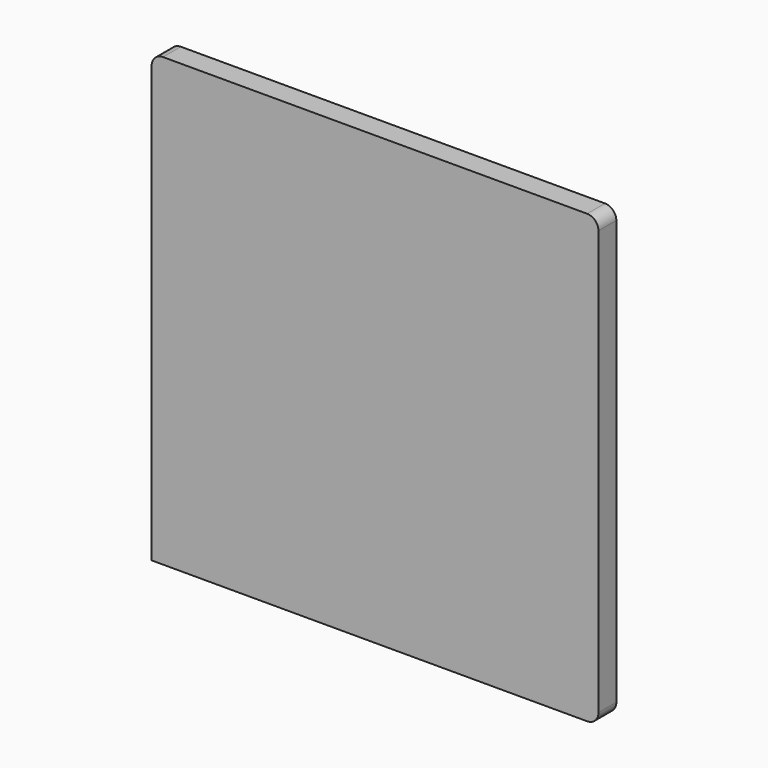
from build123d import *

# Parameters (mm, degrees)
F0_W     = 200
F0_H     = 200
F1_DEPTH = 10
F4_R     = 5.08


# Not quite as in the source:
# - the program builds the solid bodies; features that only make, move or delete a surface that nothing else refers to are left out


with BuildPart() as f1:
    # F0 (on Front) → F1 (new body)
    with BuildSketch(Plane.XZ):
        Rectangle(F0_W, F0_H)
    extrude(amount=F1_DEPTH)

    # F4
    f4_edges = [f1.edges().sort_by_distance(p)[0] for p in [
        (-100, -5, 100),
        (100, -5, -100),
        (100, -5, 100),
    ]]
    fillet(f4_edges, radius=F4_R)


solid = f1.part
